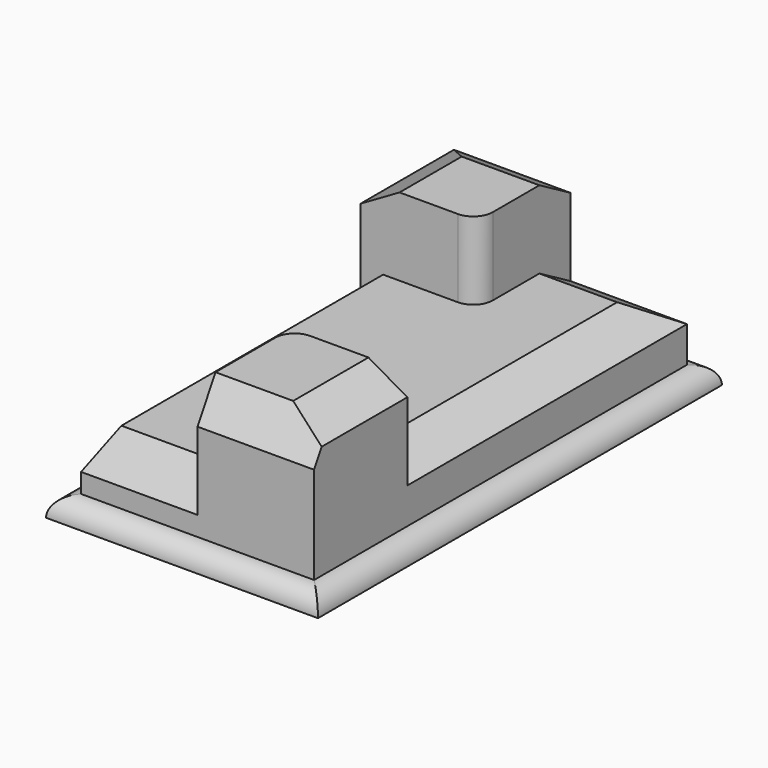
from build123d import *

# Parameters (mm, degrees)
F0_W        = 88.9
F0_H        = 165.1
F1_DEPTH    = 6.35
F2_DEPTH    = 25.4
F3_DEPTH    = 50.8
F4_R        = 6.34999
F5_C1_SIZE2 = 12.7
F5_C1_SIZE  = 7.3323484187
F5_C2_SIZE2 = 12.7
F5_C2_SIZE  = 7.3323484187
F5_C3_SIZE2 = 12.7
F5_C3_SIZE  = 7.3323484187
F5_C4_SIZE2 = 12.7
F5_C4_SIZE  = 7.3323484187
F5_C5_SIZE2 = 7.3323484187
F5_C5_SIZE  = 12.7
F5_C6_SIZE2 = 7.3323484187
F5_C6_SIZE  = 12.7
F5_C7_SIZE2 = 12.7
F5_C7_SIZE  = 7.3323484187
F5_C8_SIZE2 = 7.3323484187
F5_C8_SIZE  = 12.7


# Not quite as in the source:
# - a fillet or chamfer is up to 0.001 mm smaller than in the source, because OpenCascade refuses the exact size


with BuildPart() as f1:
    # F0 (on Top) → F1 (new body)
    with BuildSketch(Plane.XY):
        with Locations((-6.35, 1.5239301443)):
            Rectangle(F0_W, F0_H)
        Polygon((-44.45, 39.6239301443), (-44.45, 77.7239301443), (-6.35, 77.7239301443), (31.75, 77.7239301443), (31.75, -36.5760698557), (31.75, -74.6760698557), (-6.35, -74.6760698557), (-44.45, -74.6760698557), align=None, mode=Mode.SUBTRACT)
        with BuildLine():
            Line((31.75, 77.7239301443), (-6.35, 77.7239301443))
            Line((-6.35, 77.7239301443), (-6.35, 45.9739301443))
            ThreePointArc((-6.35, 45.9739301443), (-8.2098719395, 41.4838020838), (-12.7, 39.6239301443))
            Line((-12.7, 39.6239301443), (-44.45, 39.6239301443))
            Line((-44.45, 39.6239301443), (-44.45, -74.6760698557))
            Line((-44.45, -74.6760698557), (-6.35, -74.6760698557))
            Line((-6.35, -74.6760698557), (-6.35, -42.9260698557))
            ThreePointArc((-6.35, -42.9260698557), (-4.4901280605, -38.4359417952), (0, -36.5760698557))
            Line((0, -36.5760698557), (31.75, -36.5760698557))
            Line((31.75, -36.5760698557), (31.75, 77.7239301443))
        make_face()
        with BuildLine():
            Line((-6.35, 77.7239301443), (-44.45, 77.7239301443))
            Line((-44.45, 77.7239301443), (-44.45, 39.6239301443))
            Line((-44.45, 39.6239301443), (-12.7, 39.6239301443))
            ThreePointArc((-12.7, 39.6239301443), (-8.2098719395, 41.4838020838), (-6.35, 45.9739301443))
            Line((-6.35, 45.9739301443), (-6.35, 77.7239301443))
        make_face()
        with BuildLine():
            Line((31.75, -74.6760698557), (31.75, -36.5760698557))
            Line((31.75, -36.5760698557), (0, -36.5760698557))
            ThreePointArc((0, -36.5760698557), (-4.4901280605, -38.4359417952), (-6.35, -42.9260698557))
            Line((-6.35, -42.9260698557), (-6.35, -74.6760698557))
            Line((-6.35, -74.6760698557), (31.75, -74.6760698557))
        make_face()
    extrude(amount=F1_DEPTH)

    # F0 (on Top) → F2 (join)
    with BuildSketch(Plane.XY):
        with BuildLine():
            Line((31.75, 77.7239301443), (-6.35, 77.7239301443))
            Line((-6.35, 77.7239301443), (-6.35, 45.9739301443))
            ThreePointArc((-6.35, 45.9739301443), (-8.2098719395, 41.4838020838), (-12.7, 39.6239301443))
            Line((-12.7, 39.6239301443), (-44.45, 39.6239301443))
            Line((-44.45, 39.6239301443), (-44.45, -74.6760698557))
            Line((-44.45, -74.6760698557), (-6.35, -74.6760698557))
            Line((-6.35, -74.6760698557), (-6.35, -42.9260698557))
            ThreePointArc((-6.35, -42.9260698557), (-4.4901280605, -38.4359417952), (0, -36.5760698557))
            Line((0, -36.5760698557), (31.75, -36.5760698557))
            Line((31.75, -36.5760698557), (31.75, 77.7239301443))
        make_face()
    extrude(amount=F2_DEPTH)

    # F0 (on Top) → F3 (join)
    with BuildSketch(Plane.XY):
        with BuildLine():
            Line((-6.35, 77.7239301443), (-44.45, 77.7239301443))
            Line((-44.45, 77.7239301443), (-44.45, 39.6239301443))
            Line((-44.45, 39.6239301443), (-12.7, 39.6239301443))
            ThreePointArc((-12.7, 39.6239301443), (-8.2098719395, 41.4838020838), (-6.35, 45.9739301443))
            Line((-6.35, 45.9739301443), (-6.35, 77.7239301443))
        make_face()
        with BuildLine():
            Line((31.75, -74.6760698557), (31.75, -36.5760698557))
            Line((31.75, -36.5760698557), (0, -36.5760698557))
            ThreePointArc((0, -36.5760698557), (-4.4901280605, -38.4359417952), (-6.35, -42.9260698557))
            Line((-6.35, -42.9260698557), (-6.35, -74.6760698557))
            Line((-6.35, -74.6760698557), (31.75, -74.6760698557))
        make_face()
    extrude(amount=F3_DEPTH)

    # F4 (radius 6.35 in the source; OpenCascade refuses exactly that, so slightly less here)
    f4_edges = [f1.edges().sort_by_distance(p)[0] for p in [
        (38.1, 1.52393, 6.35),
        (-6.35, -81.02607, 6.35),
        (-6.35, 84.07393, 6.35),
        (-50.8, 1.52393, 6.35),
    ]]
    fillet(f4_edges, radius=F4_R)

    # F5: chamfer of 12.7 x 7.3323484187 on 8 edges, made by hand

    # F5_c1
    f5_c1_edges = [f1.edges().sort_by_distance(p)[0] for p in [
        (12.7, 77.7239301443, 25.4),
    ]]
    f5_c1_side = f1.faces().sort_by_distance((12.7, 77.7239301443, 25.2533530316))[0]
    chamfer(f5_c1_edges, length=F5_C1_SIZE, length2=F5_C1_SIZE2, reference=f5_c1_side)

    # F5_c2
    f5_c2_edges = [f1.edges().sort_by_distance(p)[0] for p in [
        (-25.4, 77.7239301443, 50.8),
    ]]
    f5_c2_side = f1.faces().sort_by_distance((-25.4, 77.7239301443, 50.6533530316))[0]
    chamfer(f5_c2_edges, length=F5_C2_SIZE, length2=F5_C2_SIZE2, reference=f5_c2_side)

    # F5_c3
    f5_c3_edges = [f1.edges().sort_by_distance(p)[0] for p in [
        (31.75, -55.6260698557, 50.8),
    ]]
    f5_c3_side = f1.faces().sort_by_distance((31.75, -55.6260698557, 50.6533530316))[0]
    chamfer(f5_c3_edges, length=F5_C3_SIZE, length2=F5_C3_SIZE2, reference=f5_c3_side)

    # F5_c4
    f5_c4_edges = [f1.edges().sort_by_distance(p)[0] for p in [
        (31.75, 14.2239301443, 25.4),
    ]]
    f5_c4_side = f1.faces().sort_by_distance((31.75, 14.2239301443, 25.2533530316))[0]
    chamfer(f5_c4_edges, length=F5_C4_SIZE, length2=F5_C4_SIZE2, reference=f5_c4_side)

    # F5_c5
    f5_c5_edges = [f1.edges().sort_by_distance(p)[0] for p in [
        (-25.4, -74.6760698557, 25.4),
    ]]
    f5_c5_side = f1.faces().sort_by_distance((-25.4, -74.6760698557, 25.2533530316))[0]
    chamfer(f5_c5_edges, length=F5_C5_SIZE, length2=F5_C5_SIZE2, reference=f5_c5_side)

    # F5_c6
    f5_c6_edges = [f1.edges().sort_by_distance(p)[0] for p in [
        (6.35, -74.6760698557, 50.8),
    ]]
    f5_c6_side = f1.faces().sort_by_distance((6.35, -74.6760698557, 50.6533530316))[0]
    chamfer(f5_c6_edges, length=F5_C6_SIZE, length2=F5_C6_SIZE2, reference=f5_c6_side)

    # F5_c7
    f5_c7_edges = [f1.edges().sort_by_distance(p)[0] for p in [
        (-44.45, 52.3239301443, 50.8),
    ]]
    f5_c7_side = f1.faces().sort_by_distance((-44.45, 52.3239301443, 50.6533530316))[0]
    chamfer(f5_c7_edges, length=F5_C7_SIZE, length2=F5_C7_SIZE2, reference=f5_c7_side)

    # F5_c8
    f5_c8_edges = [f1.edges().sort_by_distance(p)[0] for p in [
        (-44.45, -13.8598956463, 25.4),
    ]]
    f5_c8_side = f1.faces().sort_by_distance((-44.45, -13.8598956463, 25.2533530316))[0]
    chamfer(f5_c8_edges, length=F5_C8_SIZE, length2=F5_C8_SIZE2, reference=f5_c8_side)


solid = f1.part
